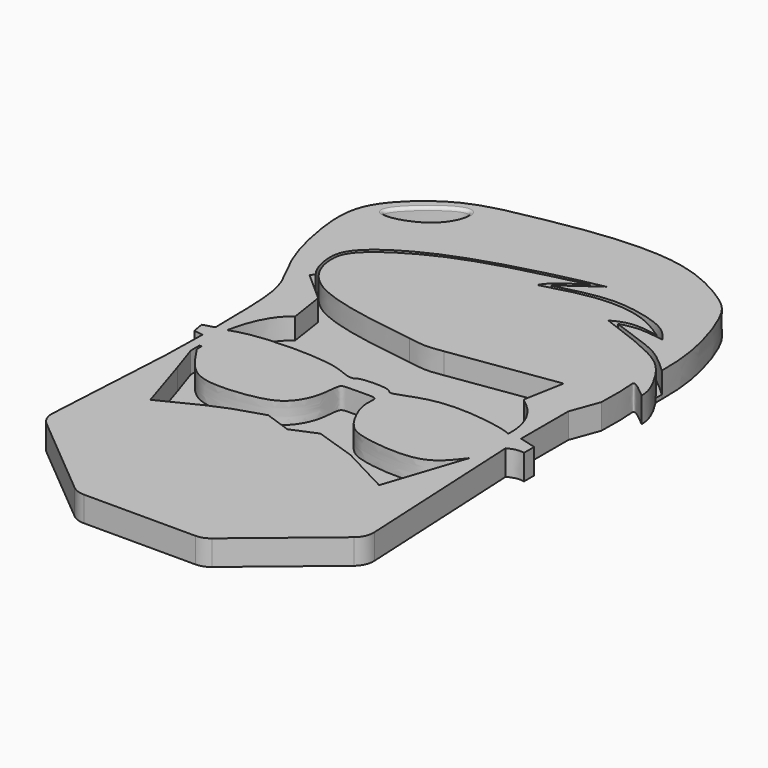
from build123d import *

# Parameters (mm, degrees)
F1_DEPTH = 2.5
F2_DEPTH = 0.4
F4_DEPTH = 25
F5_R     = 0.3
F6_R     = 2


with BuildPart() as f1:
    # F0 (on Top) → F1 (new body)
    with BuildSketch(Plane.XY):
        with BuildLine():
            Line((19.3143635988, -20.3633159399), (18.3964278549, -2.0045845304))
            add(Edge.make_bspline(
                [(19.9877452105, -1.7105005682), (19.3365439773, -1.604490797), (18.973082304, -1.7105005682), (18.3964278549, -2.0045845304)],
                knots=[0, 0, 0, 0, 1.6182633603, 1.6182633603, 1.6182633603, 1.6182633603], degree=3))
            Line((19.9877452105, -1.7105005682), (19.9877452105, -0.4535293556))
            Line((19.9877452105, -0.4535293556), (18.3272361755, 0))
            Line((18.3272361755, 0), (18.3272361755, 5.8558322489))
            Line((18.3272361755, 5.8558322489), (19.3540994078, 8.6636645719))
            add(Edge.make_bspline(
                [(21.1053676903, 11.4783952013), (20.346013658, 12.1235673859), (19.1429654278, 13.1457167679), (19.4282438149, 11.727931832), (19.3841464515, 9.9054598173), (19.3540994078, 8.6636645719)],
                knots=[0, 0, 0, 0, 0.352875749, 0.5590627392, 1, 1, 1, 1], degree=3))
            add(Edge.make_bspline(
                [(19.7057239711, 14.9584563474), (20.2432396633, 14.170375455), (21.0559924363, 12.5818666564), (21.0850616665, 11.8132536321), (21.1053676903, 11.4783952013)],
                knots=[0.6498365798, 0.6498365798, 0.6498365798, 0.6498365798, 0.8484229895, 1, 1, 1, 1], degree=3))
            add(Edge.make_bspline(
                [(11.2237641588, 19.6996759623), (13.2597408162, 18.9717113473), (16.7147629057, 17.6530628402), (18.6578334395, 16.3824862852), (19.5335411885, 15.2109028582), (19.7057239711, 14.9584563474)],
                knots=[0, 0, 0, 0, 0.3404257179, 0.5862232545, 0.6498365798, 0.6498365798, 0.6498365798, 0.6498365798], degree=3))
            add(Edge.make_bspline(
                [(15.6803019345, 20.1220028102), (13.6849842966, 20.5306820571), (12.6180816442, 20.5170344561), (11.2237641588, 19.6996759623)],
                knots=[0, 0, 0, 0, 4.476504095, 4.476504095, 4.476504095, 4.476504095], degree=3))
            add(Edge.make_bspline(
                [(3.2035578042, 20.9153220057), (5.1222645559, 21.4568261318), (8.6901300407, 22.4637616001), (13.1225299514, 21.8346379405), (14.8806506671, 20.657433983), (15.6803019345, 20.1220028102)],
                knots=[0, 0, 0, 0, 0.3881068561, 0.7216908238, 1, 1, 1, 1], degree=3))
            add(Edge.make_bspline(
                [(6.3527934253, 23.4875977039), (5.3911949508, 22.8385198861), (3.8526367862, 22.1654009074), (3.2035578042, 20.9153220057)],
                knots=[0, 0, 0, 0, 4.0662374826, 4.0662374826, 4.0662374826, 4.0662374826], degree=3))
            add(Edge.make_bspline(
                [(1.0399611201, 7.7654579654), (-2.7318884937, 8.2923337417), (-8.7734230987, 9.1362534524), (-11.7076581593, 12.0441958399), (-12.1527378029, 14.9000185552), (-10.9919886615, 16.9623718555), (-5.4907141448, 20.5170677304), (2.3236428619, 22.5755654148), (5.1824230757, 23.2226744819), (6.3527934253, 23.4875977039)],
                knots=[0, 0, 0, 0, 0.2042285334, 0.3271216719, 0.4292217838, 0.5222648989, 0.6853905786, 0.8712004733, 1, 1, 1, 1], degree=3))
            add(Edge.make_bspline(
                [(4.5257564634, 7.7173779719), (3.0833582859, 7.4769784696), (2.6179684792, 7.4824374169), (1.0399611201, 7.7654579654)],
                knots=[0, 0, 0, 0, 3.4861269141, 3.4861269141, 3.4861269141, 3.4861269141], degree=3))
            Line((4.5257564634, 7.7173779719), (15.13083186, 9.2799887061))
            Line((15.13083186, 9.2799887061), (14.3887652084, 5.2819116972))
            Line((14.3887652084, 5.2819116972), (14.5450271666, 5.1127821207))
            add(Edge.make_bspline(
                [(17.0286819339, 0), (17.1195473522, 1.4781664358), (16.7560856789, 3.5377820022), (14.5450271666, 5.1127821207)],
                knots=[0, 0, 0, 0, 5.684107847, 5.684107847, 5.684107847, 5.684107847], degree=3))
            add(Edge.make_bspline(
                [(17.0286819339, 0), (16.4532009512, 0.3574933507), (15.2719505131, 0.5089356564), (14.3027193844, 0.6906664348)],
                knots=[0, 0, 0, 0, 2.8120974281, 2.8120974281, 2.8120974281, 2.8120974281], degree=3))
            add(Edge.make_bspline(
                [(14.3027193844, 0.6906664348), (13.1674472222, 0.8568038958), (9.0476195785, 1.2869949764), (5.5375746632, -0.7015296503), (5.2701889597, 0.2628259779), (2.1729229354, 0.1424737716), (2.0773697837, -0.2153899535), (1.1423284618, -0.3029676347), (-0.5601199672, 0.8223308858), (-7.6235165642, 0.9085316585), (-9.9079050337, 0.3116322353), (-10.8367037028, 0)],
                knots=[0, 0, 0, 0, 0.16589079, 0.3002366274, 0.3572542238, 0.4776106853, 0.5170360556, 0.5766544105, 0.6778819904, 0.8674650104, 1, 1, 1, 1], degree=3))
            add(Edge.make_bspline(
                [(-10.8367037028, 0), (-10.2915121242, 2.7805704158), (-9.1708386317, 4.416147247), (-8.1410305575, 5.0522051752)],
                knots=[0, 0, 0, 0, 5.7263802562, 5.7263802562, 5.7263802562, 5.7263802562], degree=3))
            Line((-8.1410305575, 5.0522051752), (-8.676792495, 8.5916155949))
            Line((-8.676792495, 8.5916155949), (-11.6265844554, 11.2010473385))
            Line((-11.6265844554, 11.2010473385), (-11.3057242922, 11.5637587726))
            add(Edge.make_bspline(
                [(-11.3057242922, 11.5637587726), (-11.8067972362, 12.1816322207), (-12.2291309536, 13.5430680788), (-12.3249606098, 15.3319608986), (-11.1743065009, 17.2908849911), (-6.1648326672, 20.5390466802), (2.4740862367, 22.9945424637), (6.0497078202, 23.7202039732), (7.5790267438, 24.0306444466)],
                knots=[0, 0, 0, 0, 0.1244489063, 0.232945409, 0.3513627478, 0.5545720119, 0.8095320169, 1, 1, 1, 1], degree=3))
            add(Edge.make_bspline(
                [(7.5790267438, 24.0306444466), (6.4341945884, 23.1911012282), (5.1328339614, 22.373015061), (4.1445302777, 21.5120147914)],
                knots=[0, 0, 0, 0, 4.2590211687, 4.2590211687, 4.2590211687, 4.2590211687], degree=3))
            add(Edge.make_bspline(
                [(4.1445302777, 21.5120147914), (5.6646425406, 21.904039834), (8.4709887046, 22.6277745221), (11.598535238, 22.4727667915), (15.1867862848, 21.524058548), (16.1312488534, 20.3208391914), (16.5419336408, 19.7976380587)],
                knots=[0, 0, 0, 0, 0.2923280047, 0.5396795977, 0.7998368672, 1, 1, 1, 1], degree=3))
            add(Edge.make_bspline(
                [(16.5419336408, 19.7976380587), (15.6131954618, 19.9458334915), (13.9232098768, 20.2154984529), (12.6928085243, 19.8777415398), (12.1385790408, 19.7256002575)],
                knots=[0, 0, 0, 0, 0.5495539058, 1, 1, 1, 1], degree=3))
            add(Edge.make_bspline(
                [(12.1385790408, 19.7256002575), (13.5828707286, 19.2224597044), (16.0251751649, 18.3789169832), (17.7090783417, 17.5392345588), (19.039353397, 16.37127686), (19.7057239711, 15.7252270728)],
                knots=[0, 0, 0, 0, 0.405031113, 0.6763857708, 1, 1, 1, 1], degree=3))
            add(Edge.make_bspline(
                [(19.7057239711, 15.7252270728), (19.7359216256, 17.4237978573), (19.4587349529, 20.8340866663), (17.5126743126, 26.2558574723), (15.7144793044, 27.9345045661), (10.7449498819, 30.8199210878), (3.3248771542, 30.9928747097), (-3.8561393831, 29.708487922), (-9.4574870573, 28.6112378909), (-13.1704713324, 26.0755862812), (-16.1280027822, 22.6731361603), (-15.9722020506, 17.9954230117), (-14.6407943429, 12.4836944034), (-12.4309998743, 9.0554131932), (-11.885398405, 5.8668180058), (-11.8552308476, 2.039763039), (-11.8375699967, -0.2006939758)],
                knots=[0, 0, 0, 0, 0.0735509361, 0.1484847134, 0.1980689984, 0.2721735954, 0.3600547881, 0.4473786975, 0.5232275305, 0.590388971, 0.6559126102, 0.7238537006, 0.8005644768, 0.8641156898, 0.9204676942, 1, 1, 1, 1], degree=3))
            Line((-11.8375699967, -0.2006939758), (-12.9424929619, -0.5236718571))
            Line((-12.9424929619, -0.5236718571), (-12.755506672, -1.6625929857))
            Line((-12.755506672, -1.6625929857), (-11.8375699967, -1.7985836603))
            Line((-11.8375699967, -1.7985836603), (-11.9294784963, -6.2202941626))
            Line((-11.9294784963, -6.2202941626), (-12.7114243805, -20.3633159399))
            Line((-12.7114243805, -20.3633159399), (-2.9880956281, -28.4887552261))
            Line((-2.9880956281, -28.4887552261), (9.5230396837, -28.4887552261))
            Line((9.5230396837, -28.4887552261), (19.3143635988, -20.3633159399))
        make_face()
        with BuildLine():
            add(Edge.make_bspline(
                [(-10.6697911397, -3.9698407054), (-9.9129347452, -5.1360266516), (-8.5125401917, -7.293794571), (-5.6265512876, -7.9094603122), (-1.7254263057, -7.455632825), (0.4626344375, -6.5103942846), (1.7082342472, -4.1319275301), (1.694296067, -2.0135816331), (2.0561640847, -1.6906637404), (3.0756210282, -1.688037383), (4.1255565114, -1.7090215691), (4.8975466888, -1.6461018196), (5.4577601827, -1.8482663547), (5.0279175488, -3.250166887), (6.5658230074, -6.4770896752), (8.3075196101, -7.4715799481), (12.4761598744, -7.9879746696), (15.438224677, -7.3923063905), (16.645589701, -5.8225115886), (17.2429308295, -5.0458591431)],
                knots=[0, 0, 0, 0, 0.0813593087, 0.1505373195, 0.2323024389, 0.2952571348, 0.3624143346, 0.4208475821, 0.4458805968, 0.486689292, 0.53071889, 0.5671788484, 0.5935230862, 0.6394088119, 0.7160700714, 0.7751270809, 0.8589617901, 0.930221663, 1, 1, 1, 1], degree=3))
            Line((17.2429308295, -5.0458591431), (14.6127883345, -12.964874506))
            Line((14.6127883345, -12.964874506), (9.7241541371, -10.3919096291))
            Line((9.7241541371, -10.3919096291), (5.6645865552, -9.0482495725))
            Line((5.6645865552, -9.0482495725), (3.2059757505, -10.0774355233))
            Line((3.2059757505, -10.0774355233), (0.5758327316, -9.1626038775))
            Line((0.5758327316, -9.1626038775), (-2.2830176167, -10.0774355233))
            Line((-2.2830176167, -10.0774355233), (-4.2262595171, -10.8908856468))
            Line((-4.2262595171, -10.8908856468), (-8.1722484902, -12.850520201))
            Line((-8.1722484902, -12.850520201), (-9.9447350949, -7.2757625021))
            Line((-9.9447350949, -7.2757625021), (-10.8881564811, -4.4455006719))
            Line((-10.8881564811, -4.4455006719), (-10.8881564811, -3.3591378015))
            Line((-10.8881564811, -3.3591378015), (-10.6697911397, -3.3591378015))
            Line((-10.6697911397, -3.3591378015), (-10.6697911397, -3.9698407054))
        make_face(mode=Mode.SUBTRACT)
    extrude(amount=F1_DEPTH)

    # F0 (on Top) → F2 (join)
    with BuildSketch(Plane.XY):
        with BuildLine():
            add(Edge.make_bspline(
                [(11.2237641588, 19.6996759623), (13.2597408162, 18.9717113473), (16.7147629057, 17.6530628402), (18.6578334395, 16.3824862852), (19.5335411885, 15.2109028582), (19.7057239711, 14.9584563474)],
                knots=[0, 0, 0, 0, 0.3404257179, 0.5862232545, 0.6498365798, 0.6498365798, 0.6498365798, 0.6498365798], degree=3))
            Line((19.7057239711, 14.9584563474), (19.7057239711, 15.7252270728))
            add(Edge.make_bspline(
                [(12.1385790408, 19.7256002575), (13.5828707286, 19.2224597044), (16.0251751649, 18.3789169832), (17.7090783417, 17.5392345588), (19.039353397, 16.37127686), (19.7057239711, 15.7252270728)],
                knots=[0, 0, 0, 0, 0.405031113, 0.6763857708, 1, 1, 1, 1], degree=3))
            add(Edge.make_bspline(
                [(16.5419336408, 19.7976380587), (15.6131954618, 19.9458334915), (13.9232098768, 20.2154984529), (12.6928085243, 19.8777415398), (12.1385790408, 19.7256002575)],
                knots=[0, 0, 0, 0, 0.5495539058, 1, 1, 1, 1], degree=3))
            add(Edge.make_bspline(
                [(4.1445302777, 21.5120147914), (5.6646425406, 21.904039834), (8.4709887046, 22.6277745221), (11.598535238, 22.4727667915), (15.1867862848, 21.524058548), (16.1312488534, 20.3208391914), (16.5419336408, 19.7976380587)],
                knots=[0, 0, 0, 0, 0.2923280047, 0.5396795977, 0.7998368672, 1, 1, 1, 1], degree=3))
            add(Edge.make_bspline(
                [(7.5790267438, 24.0306444466), (6.4341945884, 23.1911012282), (5.1328339614, 22.373015061), (4.1445302777, 21.5120147914)],
                knots=[0, 0, 0, 0, 4.2590211687, 4.2590211687, 4.2590211687, 4.2590211687], degree=3))
            add(Edge.make_bspline(
                [(-11.3057242922, 11.5637587726), (-11.8067972362, 12.1816322207), (-12.2291309536, 13.5430680788), (-12.3249606098, 15.3319608986), (-11.1743065009, 17.2908849911), (-6.1648326672, 20.5390466802), (2.4740862367, 22.9945424637), (6.0497078202, 23.7202039732), (7.5790267438, 24.0306444466)],
                knots=[0, 0, 0, 0, 0.1244489063, 0.232945409, 0.3513627478, 0.5545720119, 0.8095320169, 1, 1, 1, 1], degree=3))
            Line((-11.3057242922, 11.5637587726), (-11.6265844554, 11.2010473385))
            Line((-11.6265844554, 11.2010473385), (-8.676792495, 8.5916155949))
            Line((-8.676792495, 8.5916155949), (-8.1410305575, 5.0522051752))
            add(Edge.make_bspline(
                [(-10.8367037028, 0), (-10.2915121242, 2.7805704158), (-9.1708386317, 4.416147247), (-8.1410305575, 5.0522051752)],
                knots=[0, 0, 0, 0, 5.7263802562, 5.7263802562, 5.7263802562, 5.7263802562], degree=3))
            add(Edge.make_bspline(
                [(14.3027193844, 0.6906664348), (13.1674472222, 0.8568038958), (9.0476195785, 1.2869949764), (5.5375746632, -0.7015296503), (5.2701889597, 0.2628259779), (2.1729229354, 0.1424737716), (2.0773697837, -0.2153899535), (1.1423284618, -0.3029676347), (-0.5601199672, 0.8223308858), (-7.6235165642, 0.9085316585), (-9.9079050337, 0.3116322353), (-10.8367037028, 0)],
                knots=[0, 0, 0, 0, 0.16589079, 0.3002366274, 0.3572542238, 0.4776106853, 0.5170360556, 0.5766544105, 0.6778819904, 0.8674650104, 1, 1, 1, 1], degree=3))
            add(Edge.make_bspline(
                [(17.0286819339, 0), (16.4532009512, 0.3574933507), (15.2719505131, 0.5089356564), (14.3027193844, 0.6906664348)],
                knots=[0, 0, 0, 0, 2.8120974281, 2.8120974281, 2.8120974281, 2.8120974281], degree=3))
            add(Edge.make_bspline(
                [(17.0286819339, 0), (17.1195473522, 1.4781664358), (16.7560856789, 3.5377820022), (14.5450271666, 5.1127821207)],
                knots=[0, 0, 0, 0, 5.684107847, 5.684107847, 5.684107847, 5.684107847], degree=3))
            Line((14.5450271666, 5.1127821207), (14.3887652084, 5.2819116972))
            Line((14.3887652084, 5.2819116972), (15.13083186, 9.2799887061))
            Line((15.13083186, 9.2799887061), (4.5257564634, 7.7173779719))
            add(Edge.make_bspline(
                [(4.5257564634, 7.7173779719), (3.0833582859, 7.4769784696), (2.6179684792, 7.4824374169), (1.0399611201, 7.7654579654)],
                knots=[0, 0, 0, 0, 3.4861269141, 3.4861269141, 3.4861269141, 3.4861269141], degree=3))
            add(Edge.make_bspline(
                [(1.0399611201, 7.7654579654), (-2.7318884937, 8.2923337417), (-8.7734230987, 9.1362534524), (-11.7076581593, 12.0441958399), (-12.1527378029, 14.9000185552), (-10.9919886615, 16.9623718555), (-5.4907141448, 20.5170677304), (2.3236428619, 22.5755654148), (5.1824230757, 23.2226744819), (6.3527934253, 23.4875977039)],
                knots=[0, 0, 0, 0, 0.2042285334, 0.3271216719, 0.4292217838, 0.5222648989, 0.6853905786, 0.8712004733, 1, 1, 1, 1], degree=3))
            add(Edge.make_bspline(
                [(6.3527934253, 23.4875977039), (5.3911949508, 22.8385198861), (3.8526367862, 22.1654009074), (3.2035578042, 20.9153220057)],
                knots=[0, 0, 0, 0, 4.0662374826, 4.0662374826, 4.0662374826, 4.0662374826], degree=3))
            add(Edge.make_bspline(
                [(3.2035578042, 20.9153220057), (5.1222645559, 21.4568261318), (8.6901300407, 22.4637616001), (13.1225299514, 21.8346379405), (14.8806506671, 20.657433983), (15.6803019345, 20.1220028102)],
                knots=[0, 0, 0, 0, 0.3881068561, 0.7216908238, 1, 1, 1, 1], degree=3))
            add(Edge.make_bspline(
                [(15.6803019345, 20.1220028102), (13.6849842966, 20.5306820571), (12.6180816442, 20.5170344561), (11.2237641588, 19.6996759623)],
                knots=[0, 0, 0, 0, 4.476504095, 4.476504095, 4.476504095, 4.476504095], degree=3))
        make_face()
        with BuildLine():
            Line((14.6127883345, -12.964874506), (17.2429308295, -5.0458591431))
            add(Edge.make_bspline(
                [(-10.6697911397, -3.9698407054), (-9.9129347452, -5.1360266516), (-8.5125401917, -7.293794571), (-5.6265512876, -7.9094603122), (-1.7254263057, -7.455632825), (0.4626344375, -6.5103942846), (1.7082342472, -4.1319275301), (1.694296067, -2.0135816331), (2.0561640847, -1.6906637404), (3.0756210282, -1.688037383), (4.1255565114, -1.7090215691), (4.8975466888, -1.6461018196), (5.4577601827, -1.8482663547), (5.0279175488, -3.250166887), (6.5658230074, -6.4770896752), (8.3075196101, -7.4715799481), (12.4761598744, -7.9879746696), (15.438224677, -7.3923063905), (16.645589701, -5.8225115886), (17.2429308295, -5.0458591431)],
                knots=[0, 0, 0, 0, 0.0813593087, 0.1505373195, 0.2323024389, 0.2952571348, 0.3624143346, 0.4208475821, 0.4458805968, 0.486689292, 0.53071889, 0.5671788484, 0.5935230862, 0.6394088119, 0.7160700714, 0.7751270809, 0.8589617901, 0.930221663, 1, 1, 1, 1], degree=3))
            Line((-10.6697911397, -3.9698407054), (-10.6697911397, -3.3591378015))
            Line((-10.6697911397, -3.3591378015), (-10.8881564811, -3.3591378015))
            Line((-10.8881564811, -3.3591378015), (-10.8881564811, -4.4455006719))
            Line((-10.8881564811, -4.4455006719), (-9.9447350949, -7.2757625021))
            Line((-9.9447350949, -7.2757625021), (-8.1722484902, -12.850520201))
            Line((-8.1722484902, -12.850520201), (-4.2262595171, -10.8908856468))
            Line((-4.2262595171, -10.8908856468), (-2.2830176167, -10.0774355233))
            Line((-2.2830176167, -10.0774355233), (0.5758327316, -9.1626038775))
            Line((0.5758327316, -9.1626038775), (3.2059757505, -10.0774355233))
            Line((3.2059757505, -10.0774355233), (5.6645865552, -9.0482495725))
            Line((5.6645865552, -9.0482495725), (9.7241541371, -10.3919096291))
            Line((9.7241541371, -10.3919096291), (14.6127883345, -12.964874506))
        make_face()
    extrude(amount=F2_DEPTH)

    # F3 (on face) → F4 (cut)
    with BuildSketch(Plane.XY.offset(2.5)):
        with BuildLine():
            add(Edge.make_bspline(
                [(-8.582255803, 27.2364169359), (-9.1235589165, 27.6345436658), (-12.2293598707, 25.6001471829), (-15.1685956444, 22.0901921647), (-8.978641791, 23.6296820418), (-8.1108859623, 26.8897259071), (-8.582255803, 27.2364169359)],
                knots=[0, 0, 0, 0, 0.2662756438, 0.4910220922, 0.7681256496, 1, 1, 1, 1], degree=3))
        make_face()
    extrude(amount=-F4_DEPTH, mode=Mode.SUBTRACT)

    # F5
    f5_edges = [f1.edges().sort_by_distance(p)[0] for p in [
        (-13.445995, 22.876664, 2.5),
        (-13.445995, 22.876664, 0),
    ]]
    fillet(f5_edges, radius=F5_R)

    # F6
    f6_edges = [f1.edges().sort_by_distance(p)[0] for p in [
        (-12.711424, -20.363316, 1.25),
        (-2.988096, -28.488755, 1.25),
        (9.52304, -28.488755, 1.25),
        (19.314364, -20.363316, 1.25),
    ]]
    fillet(f6_edges, radius=F6_R)


solid = f1.part
